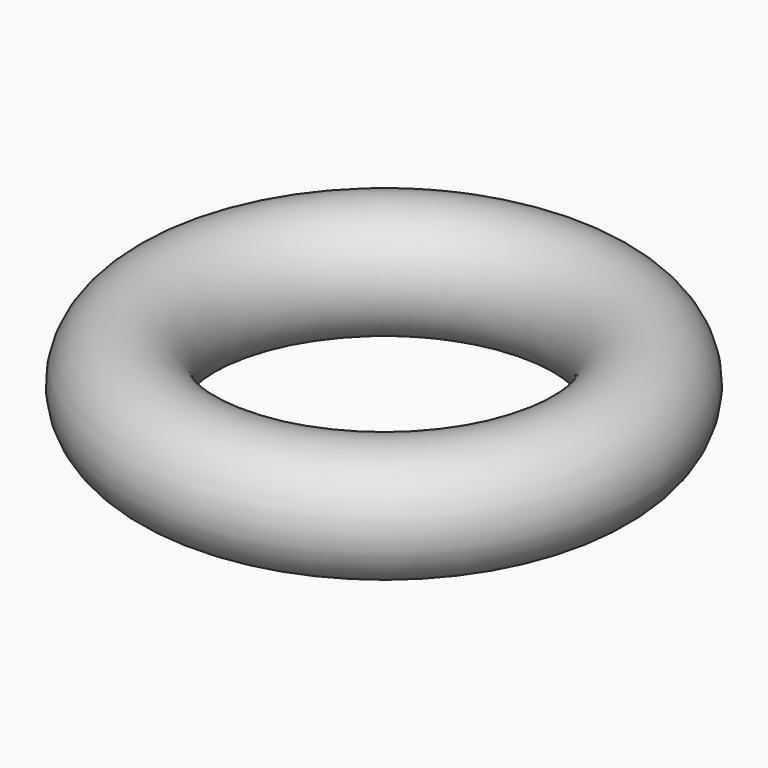
from build123d import *

# Parameters (mm, degrees)
F2_R     = 4.2022748897
F4_R     = 4
F5_DEPTH = 25
F6_DEPTH = 25


# Not quite as in the source:
# - the program builds the solid bodies; features that only make, move or delete a surface that nothing else refers to are left out


with BuildPart() as f3:
    # F2 (on Front) → F3 (revolve)
    with BuildSketch(Plane.XZ):
        with Locations((-15, 5)):
            Circle(F2_R)
    revolve(axis=Axis((0, 0, 2.5), (0, 0, -1)))

    # F4 (on Top) → F5 (cut)
    with BuildSketch(Plane.XY):
        with Locations((-10.4587538705, 18.2102846621)):
            Circle(F4_R)
    extrude(amount=F5_DEPTH, mode=Mode.SUBTRACT)

    # F4 (on Top) → F6 (cut)
    with BuildSketch(Plane.XY):
        with Locations((-10.4587538705, 18.2102846621)):
            Circle(F4_R)
    extrude(amount=F6_DEPTH, mode=Mode.SUBTRACT)


solid = f3.part
